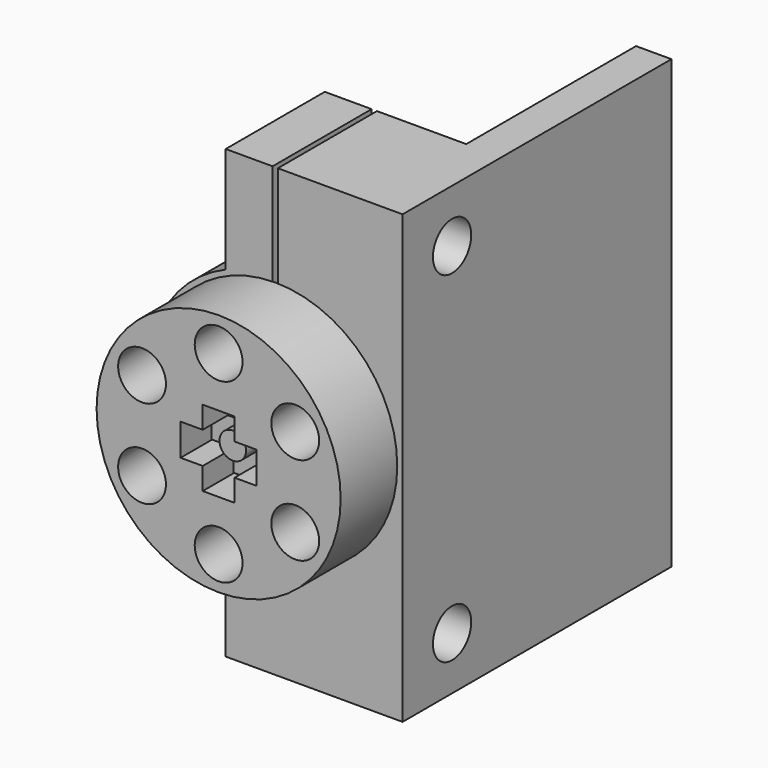
from build123d import *

# Parameters (mm, degrees)
F1_DEPTH  = 12
F2_R      = 5
F3_DEPTH  = 7
F5_DEPTH  = 2
F6_R      = 0.75
F7_DEPTH  = 1
F8_R      = 1
F9_DEPTH  = 1.8
F12_R     = 5.2
F13_DEPTH = 7
F15_DEPTH = 1.8
F17_D     = 2.7051
F18_W     = 0.3
F18_H     = 8.3822393163
F19_DEPTH = 7
F20_W     = 2
F20_H     = 25.2664991614
F21_DEPTH = 12
F23_R     = 6.9
F24_DEPTH = 4
F25_DEPTH = 4
F27_D     = 2.7051


with BuildPart() as f1:
    # F0 (on Front) → F1 (new body)
    with BuildSketch(Plane.XZ):
        with BuildLine():
            Line((3, 4), (-3, 4))
            ThreePointArc((-3, 4), (-5, 0), (-3, -4))
            Line((-3, -4), (3, -4))
            ThreePointArc((3, -4), (5, 0), (3, 4))
        make_face()
    extrude(amount=F1_DEPTH)

    # F2 (on face) → F3 (join)
    with BuildSketch(Plane.XZ.offset(12)):
        Circle(F2_R)
    extrude(amount=F3_DEPTH)

    # F4 (on face) → F5 (join)
    with BuildSketch(Plane.XZ.offset(19)):
        Polygon((0.75, 2), (-0.75, 2), (-0.75, 0.75), (-2, 0.75), (-2, -0.75), (-0.75, -0.75), (-0.75, -2), (0.75, -2), (0.75, -0.75), (2, -0.75), (2, 0.75), (0.75, 0.75), align=None)
    extrude(amount=F5_DEPTH)

    # F6 (on face) → F7 (join)
    with BuildSketch(Plane.XZ.offset(21)):
        Circle(F6_R)
    extrude(amount=F7_DEPTH)

    # F8 (on face) → F9 (join)
    with BuildSketch(Plane(origin=(0, -12, 0), x_dir=(-1, 0, 0), z_dir=(0, 1, 0))):
        with BuildLine():
            Line((-1.9, 7), (-1.9, 4))
            Line((-1.9, 4), (1.9, 4))
            Line((1.9, 4), (1.9, 7))
            ThreePointArc((1.9, 7), (0, 8.9), (-1.9, 7))
        make_face()
        with Locations((0, 7)):
            Circle(F8_R, mode=Mode.SUBTRACT)
        with BuildLine():
            Line((1.9, -4), (-1.9, -4))
            Line((-1.9, -4), (-1.9, -7))
            ThreePointArc((-1.9, -7), (0, -8.9), (1.9, -7))
            Line((1.9, -7), (1.9, -4))
        make_face()
        with Locations((0, -7)):
            Circle(F8_R, mode=Mode.SUBTRACT)
    extrude(amount=-F9_DEPTH)


with BuildPart() as f10_1:
    # F10: copy of F1
    add(f1.part)


with BuildPart() as f13:
    # F12 (on face) → F13 (new body, through all)
    with BuildSketch(Plane.XZ.offset(19)):
        with BuildLine():
            Line((7.2, -12.6332495807), (7.2, 0))
            Line((7.2, 0), (7.2, 12.6332495807))
            Line((7.2, 12.6332495807), (-2.8, 12.6332495807))
            Line((-2.8, 12.6332495807), (-2.8, 6.6332495807))
            ThreePointArc((-2.8, 6.6332495807), (-7.2, 0), (-2.8, -6.6332495807))
            Line((-2.8, -6.6332495807), (-2.8, -12.6332495807))
            Line((-2.8, -12.6332495807), (7.2, -12.6332495807))
        make_face()
        Circle(F12_R, mode=Mode.SUBTRACT)
    extrude(amount=-F13_DEPTH)

    # F14 (on face) → F15 (cut, through all)
    with BuildSketch(Plane(origin=(0, -12, 0), x_dir=(-1, 0, 0), z_dir=(0, 1, 0))):
        with BuildLine():
            Line((-2.05, 4.6249324319), (-2.05, -7))
            ThreePointArc((-2.05, -7), (0, -9.05), (2.05, -7))
            Line((2.05, -7), (2.05, 4.6541262418))
            Line((2.05, 4.6541262418), (2.05, 4.7788596966))
            Line((2.05, 4.7788596966), (2.05, 7))
            ThreePointArc((2.05, 7), (0, 9.05), (-2.05, 7))
            Line((-2.05, 7), (-2.05, 4.7788596966))
            Line((-2.05, 4.7788596966), (-2.05, 4.6249324319))
        make_face()
    extrude(amount=-F15_DEPTH, mode=Mode.SUBTRACT)

    # F17 (through all)
    with Locations(Plane(origin=(-2.8, 0, 0), x_dir=(0, -1, 0), z_dir=(-1, 0, 0))):
        with Locations((15.5, -9.6332495807), (15.5, 9.6332495807)):
            Hole(F17_D / 2)

    # F18 (on face) → F19 (cut, through all)
    with BuildSketch(Plane.XZ.offset(19)):
        with Locations((0, 8.9166247904)):
            Rectangle(F18_W, F18_H)
    extrude(amount=-F19_DEPTH, mode=Mode.SUBTRACT)

    # F20 (on face) → F21 (join, through all)
    with BuildSketch(Plane(origin=(0, -12, 0), x_dir=(-1, 0, 0), z_dir=(0, 1, 0))):
        with Locations((-6.2, 0)):
            Rectangle(F20_W, F20_H)
    extrude(amount=F21_DEPTH)


with BuildPart() as f24:
    # F23 (on face) → F24 (new body)
    with BuildSketch(Plane.XZ.offset(19)):
        Circle(F23_R)
    extrude(amount=F24_DEPTH)

    # F22 (on face) → F25 (cut, through all)
    with BuildSketch(Plane.XZ.offset(19)):
        Polygon((-0.9, 0.9), (-2.15, 0.9), (-2.15, -0.9), (-0.9, -0.9), (-0.9, -2.15), (0.9, -2.15), (0.9, -0.9), (2.15, -0.9), (2.15, 0.9), (0.9, 0.9), (0.9, 2.15), (-0.9, 2.15), align=None)
    extrude(amount=F25_DEPTH, mode=Mode.SUBTRACT)

    # F27 (through all)
    with Locations(Plane.XZ.offset(23)):
        with Locations((-4.3301270189, -2.5), (-4.3301270189, 2.5), (0, 5), (4.3301270189, 2.5), (4.3301270189, -2.5), (0, -5)):
            Hole(F27_D / 2)


solid = Compound([f1.part, f13.part, f24.part])
